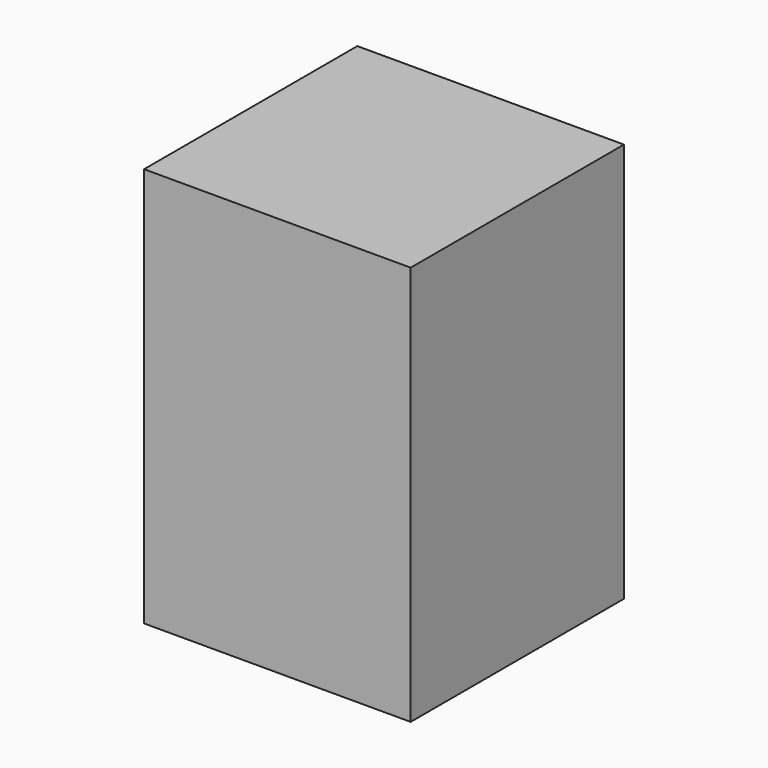
from build123d import *

# Parameters (mm, degrees)
F0_W     = 50.8
F0_H     = 76.2
F1_DEPTH = 50.8


# Not quite as in the source:
# - the program builds the solid bodies; features that only make, move or delete a surface that nothing else refers to are left out


with BuildPart() as f1:
    # F0 (on Front) → F1 (new body)
    with BuildSketch(Plane.XZ):
        with Locations((-6.5877003632, 2.022722736)):
            Rectangle(F0_W, F0_H)
    extrude(amount=F1_DEPTH)


solid = f1.part
